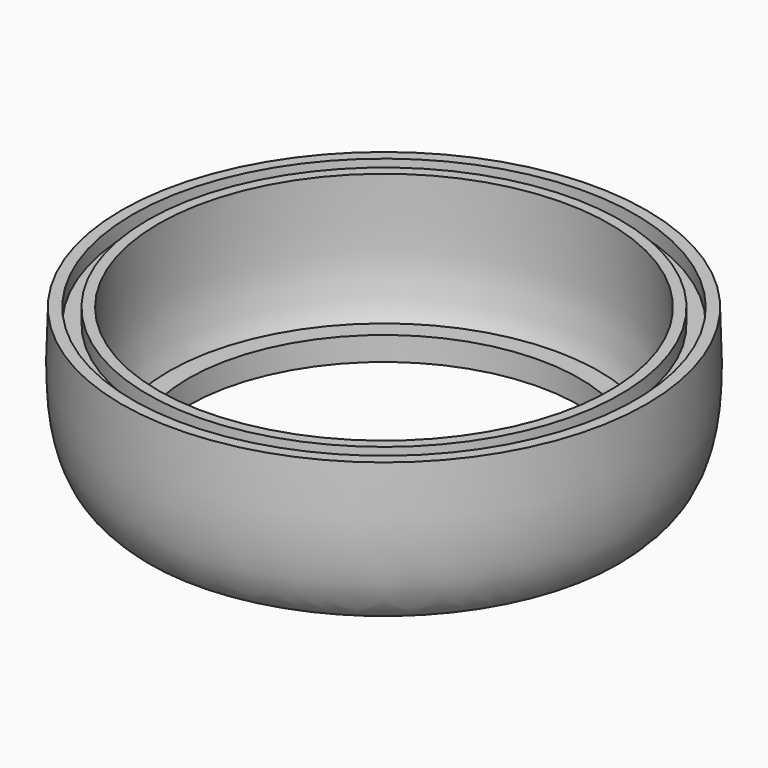
from build123d import *


with BuildPart() as f1:
    # F0 (on Front) → F1 (revolve)
    with BuildSketch(Plane.XZ):
        with BuildLine():
            Line((-26.3210460544, 0), (-26.0710460544, 0))
            Line((-26.0710460544, 0), (-26.0710460544, 1))
            Line((-26.0710460544, 1), (-26.0710460544, 3.17))
            Line((-26.0710460544, 3.17), (-28.6750581009, 3.17))
            add(Edge.make_bspline(
                [(-28.6750581009, 3.17), (-28.1018416546, 1.9161346878), (-27.3361407248, 0.8417771508), (-26.3210460544, 0)],
                knots=[0.3447375005, 0.3447375005, 0.3447375005, 0.3447375005, 0.4466613269, 0.4466613269, 0.4466613269, 0.4466613269], degree=3))
        make_face()
        with BuildLine():
            Line((-31.2336497009, 0), (-26.3210460544, 0))
            add(Edge.make_bspline(
                [(-28.6750581009, 3.17), (-28.1018416546, 1.9161346878), (-27.3361407248, 0.8417771508), (-26.3210460544, 0)],
                knots=[0.3447375005, 0.3447375005, 0.3447375005, 0.3447375005, 0.4466613269, 0.4466613269, 0.4466613269, 0.4466613269], degree=3))
            add(Edge.make_bspline(
                [(-30.0873963535, 20), (-30.3506237455, 13.7054776587), (-30.6138511374, 7.4109553174), (-28.6750581009, 3.17)],
                knots=[0, 0, 0, 0, 0.3447375005, 0.3447375005, 0.3447375005, 0.3447375005], degree=3))
            Line((-30.0873963535, 20), (-31.5, 20))
            Line((-31.5, 20), (-31.5, 18))
            Line((-31.5, 18), (-33.5, 18))
            Line((-33.5, 18), (-33.5, 20))
            Line((-33.5, 20), (-35, 20))
            add(Edge.make_bspline(
                [(-35, 20), (-35.3410522383, 11.8444622436), (-35.6821044767, 3.6889244871), (-31.2336497009, 0)],
                knots=[0, 0, 0, 0, 0.4466613269, 0.4466613269, 0.4466613269, 0.4466613269], degree=3))
        make_face()
    revolve(axis=Axis((0, 0, 10), (0, 0, 1)))


solid = f1.part
